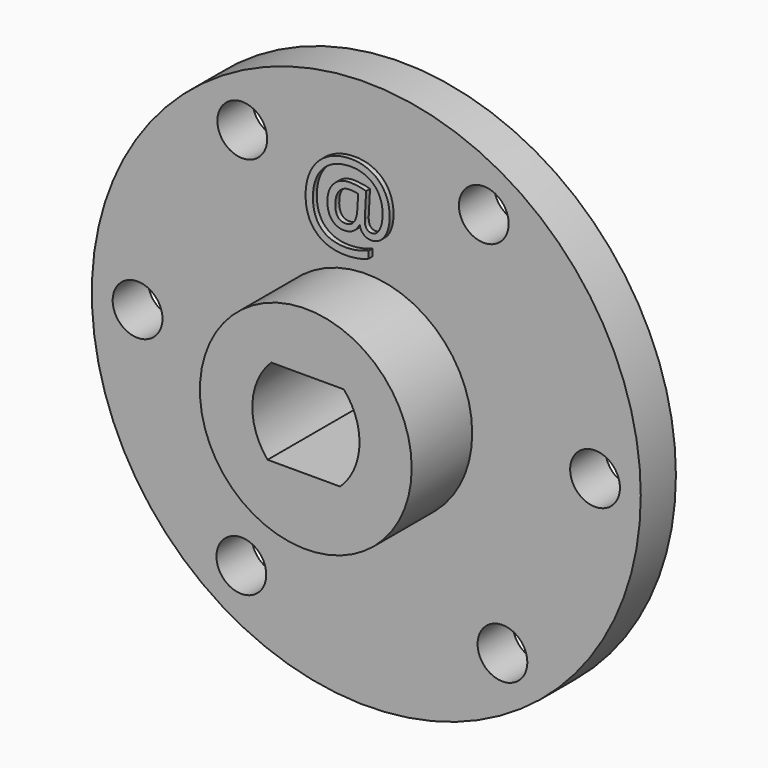
from build123d import *

# Parameters (mm, degrees)
F0_R         = 28.575
F0_R_2       = 2.5908
F0_R_3       = 11.0249222216
F1_DEPTH     = 4.572
F2_DEPTH     = 12.446
F3_TEXT_SIZE = 11.2068839371
F4_DEPTH     = 5.08


# Not quite as in the source:
# - Text() gives the source's letters only with a copy of the font that has no kerning and outlines rounded to 1/6400 em; it was checked with that copy


with BuildPart() as f1:
    # F0 (on Front) → F1 (new body)
    with BuildSketch(Plane.XZ):
        Circle(F0_R)
        with Locations((-13.0067042566, -19.9464483212)):
            Circle(F0_R_2, mode=Mode.SUBTRACT)
        with Locations((14.1729729666, -19.1353597703)):
            Circle(F0_R_2, mode=Mode.SUBTRACT)
        with Locations((-23.8125, 0)):
            Circle(F0_R_2, mode=Mode.SUBTRACT)
        with Locations((-12.9125937431, 20.0075005704)):
            Circle(F0_R_2, mode=Mode.SUBTRACT)
        Circle(F0_R_3, mode=Mode.SUBTRACT)
        with Locations((23.8125, 0)):
            Circle(F0_R_2, mode=Mode.SUBTRACT)
        with Locations((12.2324938109, 20.4304001776)):
            Circle(F0_R_2, mode=Mode.SUBTRACT)
    extrude(amount=F1_DEPTH)

    # F0 (on Front) → F2 (join)
    with BuildSketch(Plane.XZ):
        Circle(F0_R_3)
        with BuildLine():
            ThreePointArc((-3.9776887279, -4.1100203525), (-5.5602894049, 0.4815551934), (-3.6012069322, 4.9255609047))
            Line((-3.6012069322, 4.9255609047), (3.9552930678, 4.9255609047))
            ThreePointArc((3.9552930678, 4.9255609047), (5.588271517, 0.3318862891), (3.5788112721, -4.1100203525))
            Line((3.5788112721, -4.1100203525), (-3.9776887279, -4.1100203525))
        make_face(mode=Mode.SUBTRACT)
    extrude(amount=F2_DEPTH)

    # F3 (on Front) → F4 (join)
    with BuildSketch(Plane.XZ):
        with Locations((-6.5731522627, 13.3876092732)):
            Text('@', F3_TEXT_SIZE, font='Open Sans', text_align=(TextAlign.LEFT, TextAlign.BOTTOM))
    extrude(amount=F4_DEPTH)


solid = f1.part
